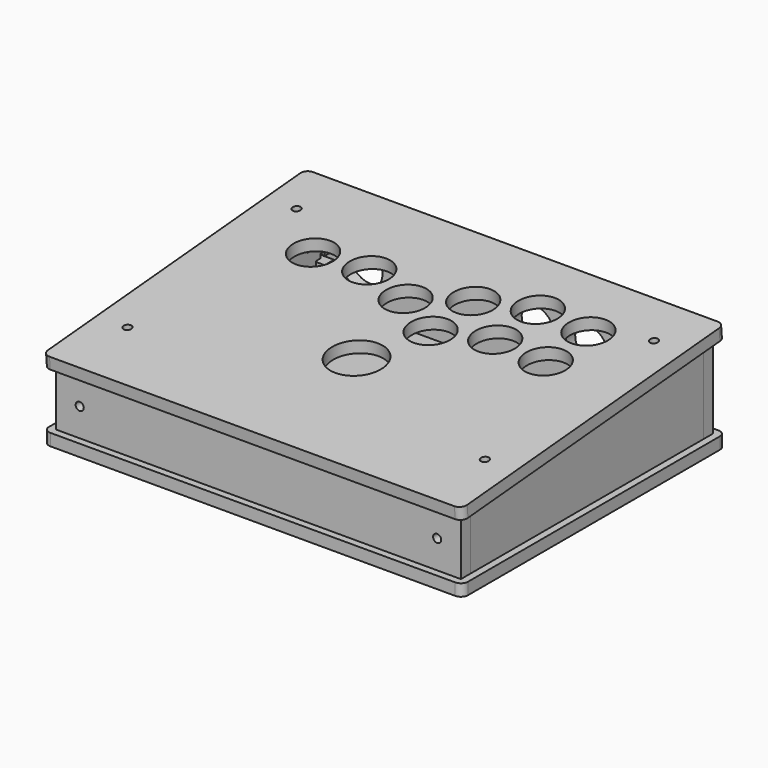
from build123d import *

# Parameters (mm, degrees)
F0_W      = 6.604
F0_H      = 4.572
F0_W_2    = 3.048
F0_W_3    = 4.572
F0_H_2    = 6.604
F0_H_3    = 3.048
F0_H_4    = 2.286
F0_W_4    = 2.286
F1_DEPTH  = 6.7056
F2_DEPTH  = 6.7056
F4_DEPTH  = 6.7056
F7_DEPTH  = 228.6
F8_R      = 2.286
F10_DEPTH = 6.7056
F9_R      = 2.286
F11_DEPTH = 6.7056
F12_W     = 228.6
F12_H     = 178.4791671152
F12_R     = 2.286
F12_R_2   = 15
F12_R_3   = 12
F12_W_2   = 6.7056
F12_H_2   = 165.0167385099
F13_DEPTH = 6.7056
F14_W     = 228.6
F14_H     = 177.8
F14_R     = 2.286
F14_W_2   = 6.7056
F14_H_2   = 164.3888
F15_DEPTH = 6.7056
F16_R     = 12
F16_R_2   = 1.6
F17_DEPTH = 6.7056


# Not quite as in the source:
# - a feature names something its author has since deleted; it is built from what else it names


with BuildPart() as f1:
    # F0 (on Right) → F1 (new body)
    with BuildSketch(Plane.YZ):
        Polygon((-82.1944, -2.286), (-82.1944, -15.875), (-56.7944, -15.875), (-56.7944, -9.271), (-59.0804, -9.271), (-59.0804, -6.223), (-56.7944, -6.223), (-56.7944, -3.175), (-52.2224, -3.175), (-52.2224, -6.223), (-49.9364, -6.223), (-49.9364, -9.271), (-52.2224, -9.271), (-52.2224, -15.875), (62.3824, -15.875), (62.3824, -9.271), (60.0964, -9.271), (60.0964, -6.223), (62.3824, -6.223), (62.3824, -3.175), (66.9544, -3.175), (66.9544, -6.223), (69.2404, -6.223), (69.2404, -9.271), (66.9544, -9.271), (66.9544, -15.875), (82.1944, -15.875), (82.1944, 5.4917421875), (75.5904, 5.4917421875), (75.5904, 3.2057421875), (72.5424, 3.2057421875), (72.5424, 5.4917421875), (69.4944, 5.4917421875), (69.4944, 10.0637421875), (72.5424, 10.0637421875), (72.5424, 12.3497421875), (75.5904, 12.3497421875), (75.5904, 10.0637421875), (82.1944, 10.0637421875), (82.1944, 30.8438203928), (67.0123928011, 29.5155668733), (67.5879693262, 22.9366970871), (69.865270406, 23.135935115), (70.1309211099, 20.0995336752), (67.8536200301, 19.9002956473), (68.119270734, 16.8638942075), (63.5646685743, 16.4654181517), (63.2990178704, 19.5018195915), (61.0217167906, 19.3025815636), (60.7560660867, 22.3389830033), (63.0333671665, 22.5382210313), (62.4577906414, 29.1170908175), (-52.3364525088, 19.0738959038), (-51.7608759837, 12.4950261176), (-49.4835749039, 12.6942641455), (-49.2179242, 9.6578627057), (-51.4952252798, 9.4586246778), (-51.2295745759, 6.422223238), (-55.7841767356, 6.0237471822), (-56.0498274395, 9.0601486219), (-58.3271285193, 8.860910594), (-58.5927792232, 11.8973120338), (-56.3154781434, 12.0965500617), (-56.8910546685, 18.6754198479), (-82.1944, 16.4616639821), (-82.1944, 2.286), (-75.5904, 2.286), (-75.5904, 4.572), (-72.5424, 4.572), (-72.5424, 2.286), (-69.4944, 2.286), (-69.4944, -2.286), (-72.5424, -2.286), (-72.5424, -4.572), (-75.5904, -4.572), (-75.5904, -2.286), align=None)
        Polygon((67.0123928011, 29.5155668733), (62.4577906414, 29.1170908175), (63.0333671665, 22.5382210313), (67.5879693262, 22.9366970871), align=None)
        Polygon((67.5879693262, 22.9366970871), (63.0333671665, 22.5382210313), (63.2990178704, 19.5018195915), (67.8536200301, 19.9002956473), align=None)
        Polygon((67.8536200301, 19.9002956473), (63.2990178704, 19.5018195915), (63.5646685743, 16.4654181517), (68.119270734, 16.8638942075), align=None)
        Polygon((-52.3364525088, 19.0738959038), (-56.8910546685, 18.6754198479), (-56.3154781434, 12.0965500617), (-51.7608759837, 12.4950261176), align=None)
        Polygon((-51.7608759837, 12.4950261176), (-56.3154781434, 12.0965500617), (-56.0498274395, 9.0601486219), (-51.4952252798, 9.4586246778), align=None)
        Polygon((-51.4952252798, 9.4586246778), (-56.0498274395, 9.0601486219), (-55.7841767356, 6.0237471822), (-51.2295745759, 6.422223238), align=None)
        with Locations((-78.8924, 0)):
            Rectangle(F0_W, F0_H)
        with Locations((-74.0664, 0)):
            Rectangle(F0_W_2, F0_H)
        with Locations((-71.0184, 0)):
            Rectangle(F0_W_2, F0_H)
        with Locations((-54.5084, -12.573)):
            Rectangle(F0_W_3, F0_H_2)
        with Locations((-54.5084, -7.747)):
            Rectangle(F0_W_3, F0_H_3)
        with Locations((-54.5084, -4.699)):
            Rectangle(F0_W_3, F0_H_3)
        with Locations((64.6684, -12.573)):
            Rectangle(F0_W_3, F0_H_2)
        with Locations((64.6684, -7.747)):
            Rectangle(F0_W_3, F0_H_3)
        with Locations((64.6684, -4.699)):
            Rectangle(F0_W_3, F0_H_3)
        with Locations((78.8924, 7.7777421875)):
            Rectangle(F0_W, F0_H)
        with Locations((74.0664, 7.7777421875)):
            Rectangle(F0_W_2, F0_H)
        with Locations((71.0184, 7.7777421875)):
            Rectangle(F0_W_2, F0_H)
        Polygon((63.2990178704, 19.5018195915), (63.0333671665, 22.5382210313), (60.7560660867, 22.3389830033), (61.0217167906, 19.3025815636), align=None)
        Polygon((69.865270406, 23.135935115), (67.5879693262, 22.9366970871), (67.8536200301, 19.9002956473), (70.1309211099, 20.0995336752), align=None)
        with Locations((74.0664, 4.3487421875)):
            Rectangle(F0_W_2, F0_H_4)
        with Locations((74.0664, 11.2067421875)):
            Rectangle(F0_W_2, F0_H_4)
        with Locations((68.0974, -7.747)):
            Rectangle(F0_W_4, F0_H_3)
        with Locations((61.2394, -7.747)):
            Rectangle(F0_W_4, F0_H_3)
        with Locations((-51.0794, -7.747)):
            Rectangle(F0_W_4, F0_H_3)
        with Locations((-57.9374, -7.747)):
            Rectangle(F0_W_4, F0_H_3)
        with Locations((-74.0664, -3.429)):
            Rectangle(F0_W_2, F0_H_4)
        with Locations((-74.0664, 3.429)):
            Rectangle(F0_W_2, F0_H_4)
        Polygon((-56.0498274395, 9.0601486219), (-56.3154781434, 12.0965500617), (-58.5927792232, 11.8973120338), (-58.3271285193, 8.860910594), align=None)
        Polygon((-49.4835749039, 12.6942641455), (-51.7608759837, 12.4950261176), (-51.4952252798, 9.4586246778), (-49.2179242, 9.6578627057), align=None)
    extrude(amount=-F1_DEPTH)


with BuildPart() as f2:
    # F0 (on Right) → F2 (new body)
    with BuildSketch(Plane.YZ):
        Polygon((-82.1944, -2.286), (-82.1944, -15.875), (-56.7944, -15.875), (-56.7944, -9.271), (-59.0804, -9.271), (-59.0804, -6.223), (-56.7944, -6.223), (-56.7944, -3.175), (-52.2224, -3.175), (-52.2224, -6.223), (-49.9364, -6.223), (-49.9364, -9.271), (-52.2224, -9.271), (-52.2224, -15.875), (62.3824, -15.875), (62.3824, -9.271), (60.0964, -9.271), (60.0964, -6.223), (62.3824, -6.223), (62.3824, -3.175), (66.9544, -3.175), (66.9544, -6.223), (69.2404, -6.223), (69.2404, -9.271), (66.9544, -9.271), (66.9544, -15.875), (82.1944, -15.875), (82.1944, 5.4917421875), (75.5904, 5.4917421875), (75.5904, 3.2057421875), (72.5424, 3.2057421875), (72.5424, 5.4917421875), (69.4944, 5.4917421875), (69.4944, 10.0637421875), (72.5424, 10.0637421875), (72.5424, 12.3497421875), (75.5904, 12.3497421875), (75.5904, 10.0637421875), (82.1944, 10.0637421875), (82.1944, 30.8438203928), (67.0123928011, 29.5155668733), (67.5879693262, 22.9366970871), (69.865270406, 23.135935115), (70.1309211099, 20.0995336752), (67.8536200301, 19.9002956473), (68.119270734, 16.8638942075), (63.5646685743, 16.4654181517), (63.2990178704, 19.5018195915), (61.0217167906, 19.3025815636), (60.7560660867, 22.3389830033), (63.0333671665, 22.5382210313), (62.4577906414, 29.1170908175), (-52.3364525088, 19.0738959038), (-51.7608759837, 12.4950261176), (-49.4835749039, 12.6942641455), (-49.2179242, 9.6578627057), (-51.4952252798, 9.4586246778), (-51.2295745759, 6.422223238), (-55.7841767356, 6.0237471822), (-56.0498274395, 9.0601486219), (-58.3271285193, 8.860910594), (-58.5927792232, 11.8973120338), (-56.3154781434, 12.0965500617), (-56.8910546685, 18.6754198479), (-82.1944, 16.4616639821), (-82.1944, 2.286), (-75.5904, 2.286), (-75.5904, 4.572), (-72.5424, 4.572), (-72.5424, 2.286), (-69.4944, 2.286), (-69.4944, -2.286), (-72.5424, -2.286), (-72.5424, -4.572), (-75.5904, -4.572), (-75.5904, -2.286), align=None)
    extrude(amount=-F2_DEPTH)


with BuildPart() as f2_1:
    # F3: moved
    add(f2.part.moved(Location((-6.7056, 0, 0))))


with BuildPart() as f4:
    # F4 (new): a face of the model
    f4_faces = [f2_1.part.faces().sort_by_distance(p)[0] for p in [
        (-13.4112, 5.0847963051, 4.1113233395),
    ]]
    extrude(f4_faces, amount=F4_DEPTH)


with BuildPart() as f5_1:
    # F5: instance of F1
    add(f1.part.mirror(Plane.YZ))


with BuildPart() as f5_2:
    # F5: instance of F2
    add(f2_1.part.mirror(Plane.YZ))


with BuildPart() as f5_3:
    # F5: instance of F4
    add(f4.part.mirror(Plane.YZ))


with BuildPart() as f5_1_1:
    # F6: moved
    add(f5_1.part.moved(Location((-228.6, 0, 0))))


with BuildPart() as f5_2_1:
    # F6: moved
    add(f5_2.part.moved(Location((-228.6, 0, 0))))


with BuildPart() as f5_3_1:
    # F6: moved
    add(f5_3.part.moved(Location((-228.6, 0, 0))))


with BuildPart() as f7:
    # F0 (on Right) → F7 (new body, through all)
    with BuildSketch(Plane.YZ):
        Polygon((-88.9, 15.875), (-88.9, -15.875), (-82.1944, -15.875), (-82.1944, -2.286), (-82.1944, 2.286), (-82.1944, 16.4616639821), align=None)
    extrude(amount=-F7_DEPTH)

    # F8 (on face) → F10 (cut, through all)
    with BuildSketch(Plane(origin=(0, -82.1944, 0), x_dir=(-1, 0, 0), z_dir=(0, 1, 0))):
        with Locations((215.1888, 0)):
            Circle(F8_R)
        with Locations((13.4112, 0)):
            Circle(F8_R)
    extrude(amount=-F10_DEPTH, mode=Mode.SUBTRACT)


with BuildPart() as f7b:
    # F0 (on Right) → F7, piece 2 (new body, through all)
    with BuildSketch(Plane.YZ):
        Polygon((82.1944, 5.4917421875), (82.1944, -15.875), (88.9, -15.875), (88.9, 31.4304843749), (82.1944, 30.8438203928), (82.1944, 10.0637421875), align=None)
    extrude(amount=-F7_DEPTH)

    # F9 (on face) → F11 (cut, through all)
    with BuildSketch(Plane.XZ.offset(-82.1944)):
        with Locations((-215.1888, 7.7777421875)):
            Circle(F9_R)
        with Locations((-13.4112, 7.7777421875)):
            Circle(F9_R)
    extrude(amount=-F11_DEPTH, mode=Mode.SUBTRACT)

    # F16 (on face) → F17 (cut, through all)
    with BuildSketch(Plane(origin=(0, 88.9, 0), x_dir=(-1, 0, 0), z_dir=(0, 1, 0))):
        with Locations((35.5112, 7.7777421875)):
            Circle(F16_R)
        with Locations((65.7112, 7.7777421875)):
            Circle(F16_R)
        with Locations((193.0888, 7.7777421875)):
            Circle(F16_R)
        with Locations((95.9112, 7.7777421875)):
            Circle(F16_R)
        with Locations((205.0888, 17.2777421875)):
            Circle(F16_R_2)
        with Locations((181.0888, -1.7222578125)):
            Circle(F16_R_2)
    extrude(amount=-F17_DEPTH, mode=Mode.SUBTRACT)


with BuildPart() as f13:
    # F12 (on face) → F13 (new body)
    with BuildSketch(Plane(origin=(0, -2.0536277888, 23.4730730368), x_dir=(1, 0, 0), z_dir=(0, -0.0871557427, 0.9961946981))):
        with BuildLine():
            ThreePointArc((-228.6, 95.301055871), (-231.4284271247, 94.1294829957), (-232.6, 91.301055871))
            Line((-232.6, 91.301055871), (-232.6, -87.1781112442))
            ThreePointArc((-232.6, -87.1781112442), (-231.4284271247, -90.006538369), (-228.6, -91.1781112442))
            Line((-228.6, -91.1781112442), (0, -91.1781112442))
            ThreePointArc((0, -91.1781112442), (2.8284271247, -90.006538369), (4, -87.1781112442))
            Line((4, -87.1781112442), (4, 91.301055871))
            ThreePointArc((4, 91.301055871), (2.8284271247, 94.1294829957), (0, 95.301055871))
            Line((0, 95.301055871), (-228.6, 95.301055871))
        make_face()
        with Locations((-114.3, 2.0614723134)):
            Rectangle(F12_W, F12_H, mode=Mode.SUBTRACT)
        Polygon((0, 91.301055871), (-228.6, 91.301055871), (-228.6, -87.1781112442), (0, -87.1781112442), (0, -80.4468969416), (-6.7056, -80.4468969416), (-6.7056, 84.5698415683), (0, 84.5698415683), align=None)
        with Locations((-215.1888, -52.7608969416)):
            Circle(F12_R, mode=Mode.SUBTRACT)
        with Locations((-13.4112, -52.7608969416)):
            Circle(F12_R, mode=Mode.SUBTRACT)
        with Locations((-114.3, -17.0817187308)):
            Circle(F12_R_2, mode=Mode.SUBTRACT)
        with Locations((-186.0070012111, 42.0698415683)):
            Circle(F12_R_3, mode=Mode.SUBTRACT)
        with Locations((-155.8732991485, 44.0698415683)):
            Circle(F12_R_3, mode=Mode.SUBTRACT)
        with Locations((-127.3769835971, 34.0698415683)):
            Circle(F12_R_3, mode=Mode.SUBTRACT)
        with Locations((-215.1888, 67.0438415683)):
            Circle(F12_R, mode=Mode.SUBTRACT)
        with Locations((-101.2230164029, 18.9698415683)):
            Circle(F12_R_3, mode=Mode.SUBTRACT)
        with Locations((-72.7267008515, 28.9698415683)):
            Circle(F12_R_3, mode=Mode.SUBTRACT)
        with Locations((-42.5929987889, 26.9698415683)):
            Circle(F12_R_3, mode=Mode.SUBTRACT)
        with Locations((-101.2230164029, 49.1698415683)):
            Circle(F12_R_3, mode=Mode.SUBTRACT)
        with Locations((-72.7267008515, 59.1698415683)):
            Circle(F12_R_3, mode=Mode.SUBTRACT)
        with Locations((-42.5929987889, 57.1698415683)):
            Circle(F12_R_3, mode=Mode.SUBTRACT)
        with Locations((-13.4112, 67.0438415683)):
            Circle(F12_R, mode=Mode.SUBTRACT)
        with Locations((-3.3528, 2.0614723134)):
            Rectangle(F12_W_2, F12_H_2)
    extrude(amount=F13_DEPTH)


with BuildPart() as f15:
    # F14 (on face) → F15 (new body)
    with BuildSketch(Plane(origin=(0, 0, -15.875), x_dir=(1, 0, 0), z_dir=(0, 0, -1))):
        with BuildLine():
            ThreePointArc((-228.6, 92.9), (-231.4284271247, 91.7284271247), (-232.6, 88.9))
            Line((-232.6, 88.9), (-232.6, -88.9))
            ThreePointArc((-232.6, -88.9), (-231.4284271247, -91.7284271247), (-228.6, -92.9))
            Line((-228.6, -92.9), (0, -92.9))
            ThreePointArc((0, -92.9), (2.8284271247, -91.7284271247), (4, -88.9))
            Line((4, -88.9), (4, 88.9))
            ThreePointArc((4, 88.9), (2.8284271247, 91.7284271247), (0, 92.9))
            Line((0, 92.9), (-228.6, 92.9))
        make_face()
        with Locations((-114.3, 0)):
            Rectangle(F14_W, F14_H, mode=Mode.SUBTRACT)
        Polygon((0, 82.1944), (0, 88.9), (-228.6, 88.9), (-228.6, -88.9), (0, -88.9), (0, -82.1944), (-6.7056, -82.1944), (-6.7056, 82.1944), align=None)
        with Locations((-215.1888, -64.6684)):
            Circle(F14_R, mode=Mode.SUBTRACT)
        with Locations((-13.4112, -64.6684)):
            Circle(F14_R, mode=Mode.SUBTRACT)
        with Locations((-215.1888, 54.5084)):
            Circle(F14_R, mode=Mode.SUBTRACT)
        with Locations((-13.4112, 54.5084)):
            Circle(F14_R, mode=Mode.SUBTRACT)
        with Locations((-3.3528, 0)):
            Rectangle(F14_W_2, F14_H_2)
    extrude(amount=F15_DEPTH)


solid = Compound([f1.part, f2_1.part, f4.part, f5_1_1.part, f5_2_1.part, f5_3_1.part, f7.part, f7b.part, f13.part, f15.part])
